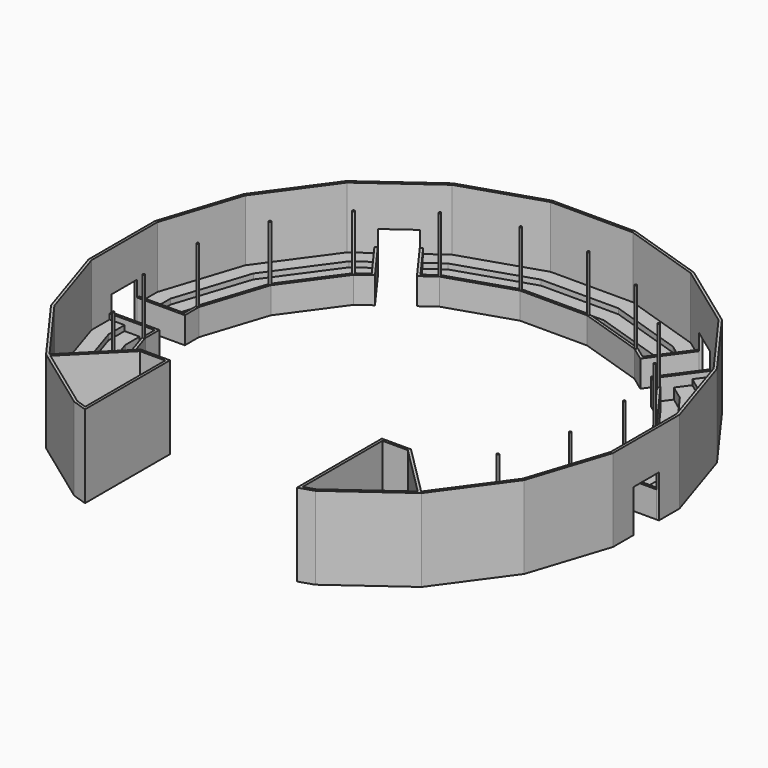
from build123d import *

# Parameters (mm, degrees)
F0_W     = 152.4
F0_H     = 1828.8
F1_DEPTH = 4754.88
F0_R     = 60.96
F2_DEPTH = 1524
F3_DEPTH = 914.4
F4_DEPTH = 1219.2
F5_DEPTH = 304.8
F6_DEPTH = 4724.4
F7_DEPTH = 2438.4


# Not quite as in the source:
# - a feature names something its author has since deleted; it is built from what else it names


with BuildPart() as f1:
    # F0 (on Top) → F1 (new body)
    with BuildSketch(Plane.XY):
        Polygon((2389.6410818405, 15087.6), (-2389.6410818405, 15087.6), (-6935.0085268224, 13610.7205905095), (-8128.5036328315, 12743.5956390277), (-8038.9251603821, 12620.301449085), (-7915.6309704393, 12709.8799215343), (-6864.9579356424, 13473.2385643428), (-2365.503293135, 14935.2), (2365.503293135, 14935.2), (6864.9579356424, 13473.2385643428), (7915.6309704393, 12709.8799215343), (8038.9251603821, 12620.301449085), (8128.5036328314, 12743.5956390277), (6935.0085268224, 13610.7205905095), align=None)
        Polygon((-14935.2, -914.4), (-15087.6, -914.4), (-15087.6, -2389.6410818405), (-13610.7205905095, -6935.0085268224), (-10801.5290181534, -10801.5290181534), (-6935.0085268224, -13610.7205905095), (-6096, -13883.3309861815), (-6096, -7924.8), (-6096, -7772.4), (-6705.6, -7772.4), (-7772.4, -7772.4), (-8728.5082974977, -8728.5082974977), (-8837.6146512164, -8837.6146512164), (-9455.8839889558, -9455.8839889558), (-10074.1533266953, -10074.1533266953), (-10692.4226644347, -10692.4226644347), (-13473.2385643428, -6864.9579356424), (-14935.2, -2365.503293135), (-14935.2, -1066.8), align=None)
        Polygon((-6248.4, -13673.5703815017), (-6864.9579356424, -13473.2385643428), (-10567.5915969054, -10783.117743811), (-7709.2738530943, -7924.8), (-6248.4, -7924.8), align=None, mode=Mode.SUBTRACT)
        Polygon((-14935.2, 914.4), (-15087.6, 914.4), (-15087.6, 0), (-15087.6, -914.4), (-14935.2, -914.4), align=None)
        Polygon((-9565.5489102916, 11511.1443705127), (-9655.127382741, 11634.4385604554), (-10801.5290181534, 10801.5290181534), (-13610.7205905095, 6935.0085268224), (-15087.6, 2389.6410818405), (-15087.6, 914.4), (-14935.2, 914.4), (-14935.2, 1066.8), (-14935.2, 2365.503293135), (-13473.2385643428, 6864.9579356424), (-10692.4226644347, 10692.4226644347), (-9688.8431002343, 11421.5658980633), align=None)
        Polygon((-8038.9251603821, 12620.301449085), (-8128.5036328315, 12743.5956390277), (-9655.127382741, 11634.4385604554), (-9565.5489102916, 11511.1443705127), align=None)
        Polygon((9608.0339121444, 11668.6539696352), (8128.5036328315, 12743.5956390277), (8038.9251603821, 12620.301449085), (9518.455439695, 11545.3597796925), align=None)
        Polygon((10801.5290181534, 10801.5290181534), (9608.0339121444, 11668.6539696352), (9518.455439695, 11545.3597796925), (9641.7496296377, 11455.7813072431), (10692.4226644347, 10692.4226644347), (13473.2385643428, 6864.9579356424), (14935.2, 2365.503293135), (14935.2, 1066.8), (14935.2, 914.4), (15087.6, 914.4), (15087.6, 2389.6410818405), (13610.7205905095, 6935.0085268224), align=None)
        with Locations((15011.4, 0)):
            Rectangle(F0_W, F0_H)
        Polygon((15087.6, -2389.6410818405), (15087.6, -914.4), (14935.2, -914.4), (14935.2, -1066.8), (14935.2, -2365.503293135), (13473.2385643428, -6864.9579356424), (10692.4226644347, -10692.4226644347), (10074.1533266953, -10074.1533266953), (9455.8839889558, -9455.8839889558), (8837.6146512164, -8837.6146512164), (8728.5082974977, -8728.5082974977), (7772.4, -7772.4), (6705.6, -7772.4), (6096, -7772.4), (6096, -13883.3309861815), (6935.0085268224, -13610.7205905095), (10801.5290181534, -10801.5290181534), (13610.7205905095, -6935.0085268224), align=None)
        Polygon((6248.4, -7924.8), (7709.2738530943, -7924.8), (10567.5915969054, -10783.117743811), (6864.9579356424, -13473.2385643428), (6248.4, -13673.5703815017), align=None, mode=Mode.SUBTRACT)
    extrude(amount=F1_DEPTH)

    # F0 (on Top) → F7 (cut)
    with BuildSketch(Plane.XY):
        Polygon((-14935.2, 914.4), (-15087.6, 914.4), (-15087.6, 0), (-15087.6, -914.4), (-14935.2, -914.4), align=None)
        Polygon((-8038.9251603821, 12620.301449085), (-8128.5036328315, 12743.5956390277), (-9655.127382741, 11634.4385604554), (-9565.5489102916, 11511.1443705127), align=None)
        Polygon((9608.0339121444, 11668.6539696352), (8128.5036328315, 12743.5956390277), (8038.9251603821, 12620.301449085), (9518.455439695, 11545.3597796925), align=None)
        with Locations((15011.4, 0)):
            Rectangle(F0_W, F0_H)
    extrude(amount=F7_DEPTH, mode=Mode.SUBTRACT)


with BuildPart() as f2:
    # F0 (on Top) → F2 (new body)
    with BuildSketch(Plane.XY):
        Polygon((-7953.1364062029, 9291.8489515433), (-9565.5489102916, 11511.1443705127), (-9688.8431002343, 11421.5658980633), (-9181.2317563546, 10722.8988217211), (-8673.6204124748, 10024.2317453789), (-8166.009068595, 9325.5646690367), (-8837.6146512164, 8837.6146512164), (-11136.0441195078, 5674.097885582), (-12344.4, 1955.1608851422), (-12344.4, 1066.8), (-13208, 1066.8), (-14071.6, 1066.8), (-14935.2, 1066.8), (-14935.2, 914.4), (-12192, 914.4), (-12192, 1931.0230964367), (-10998.562093341, 5604.047294402), (-8728.5082974977, 8728.5082974977), align=None)
        with Locations((-12268.2, 1943.0919907895)):
            Circle(F0_R, mode=Mode.SUBTRACT)
        with Locations((-11067.3031064244, 5639.072589992)):
            Circle(F0_R, mode=Mode.SUBTRACT)
        with Locations((-8783.0614743571, 8783.0614743571)):
            Circle(F0_R, mode=Mode.SUBTRACT)
    extrude(amount=F2_DEPTH)

    # F0 (on Top) → F3, piece 2 (join)
    with BuildSketch(Plane.XY):
        Polygon((-8673.6204124748, 10024.2317453789), (-9181.2317563546, 10722.8988217211), (-10074.1533266953, 10074.1533266953), (-12694.1737493978, 6468.0045856223), (-14071.6, 2228.7224904707), (-14071.6, 1066.8), (-13208, 1066.8), (-13208, 2091.9416878065), (-11915.1089344528, 6071.0512356021), (-9455.8839889558, 9455.8839889558), align=None)
    extrude(amount=F3_DEPTH)

    # F0 (on Top) → F4 (join)
    with BuildSketch(Plane.XY):
        Polygon((-9181.2317563546, 10722.8988217211), (-9688.8431002343, 11421.5658980633), (-10692.4226644347, 10692.4226644347), (-13473.2385643428, 6864.9579356424), (-14935.2, 2365.503293135), (-14935.2, 1066.8), (-14071.6, 1066.8), (-14071.6, 2228.7224904707), (-12694.1737493978, 6468.0045856223), (-10074.1533266953, 10074.1533266953), align=None)
    extrude(amount=F4_DEPTH)

    # F0 (on Top) → F5, piece 2 (join)
    with BuildSketch(Plane.XY):
        Polygon((-8166.009068595, 9325.5646690367), (-8673.6204124748, 10024.2317453789), (-9455.8839889558, 9455.8839889558), (-11915.1089344528, 6071.0512356021), (-13208, 2091.9416878065), (-13208, 1066.8), (-12344.4, 1066.8), (-12344.4, 1955.1608851422), (-11136.0441195078, 5674.097885582), (-8837.6146512164, 8837.6146512164), align=None)
    extrude(amount=F5_DEPTH)

    # F0 (on Top) → F6, piece 2 (join)
    with BuildSketch(Plane.XY):
        with Locations((-12268.2, 1943.0919907895)):
            Circle(F0_R)
        with Locations((-11067.3031064244, 5639.072589992)):
            Circle(F0_R)
        with Locations((-8783.0614743571, 8783.0614743571)):
            Circle(F0_R)
    extrude(amount=F6_DEPTH)


with BuildPart() as f2b:
    # F0 (on Top) → F2, piece 2 (new body)
    with BuildSketch(Plane.XY):
        Polygon((-7915.6309704393, 12709.8799215343), (-8038.9251603821, 12620.301449085), (-6426.5126562934, 10401.0060301156), (-5604.047294402, 10998.562093341), (-1931.0230964367, 12192), (0, 12192), (0, 12344.4), (-1955.1608851422, 12344.4), (-5674.097885582, 11136.0441195078), (-6392.7969388, 10613.8786925077), (-6900.4082826798, 11312.5457688499), (-7408.0196265596, 12011.2128451921), align=None)
        with Locations((-5639.072589992, 11067.3031064244)):
            Circle(F0_R, mode=Mode.SUBTRACT)
        with Locations((-1943.0919907895, 12268.2)):
            Circle(F0_R, mode=Mode.SUBTRACT)
        Polygon((6426.5126562934, 10401.0060301156), (8038.9251603821, 12620.301449085), (7915.6309704393, 12709.8799215343), (7408.0196265596, 12011.2128451921), (6900.4082826798, 11312.5457688499), (6392.7969388, 10613.8786925077), (5674.097885582, 11136.0441195078), (1955.1608851422, 12344.4), (0, 12344.4), (0, 12192), (1931.0230964367, 12192), (5604.047294402, 10998.562093341), align=None)
        with Locations((5639.072589992, 11067.3031064244)):
            Circle(F0_R, mode=Mode.SUBTRACT)
        with Locations((1943.0919907895, 12268.2)):
            Circle(F0_R, mode=Mode.SUBTRACT)
    extrude(amount=F2_DEPTH)

    # F0 (on Top) → F3, piece 3 (join)
    with BuildSketch(Plane.XY):
        Polygon((-6468.0045856223, 12694.1737493978), (-7408.0196265596, 12011.2128451921), (-6900.4082826798, 11312.5457688499), (-6071.0512356021, 11915.1089344528), (-2091.9416878065, 13208), (2091.9416878065, 13208), (6071.0512356021, 11915.1089344528), (6900.4082826798, 11312.5457688499), (7408.0196265596, 12011.2128451921), (6468.0045856223, 12694.1737493978), (2228.7224904707, 14071.6), (-2228.7224904707, 14071.6), align=None)
    extrude(amount=F3_DEPTH)

    # F0 (on Top) → F4, piece 3 (join)
    with BuildSketch(Plane.XY):
        Polygon((-6864.9579356424, 13473.2385643428), (-7915.6309704393, 12709.8799215343), (-7408.0196265596, 12011.2128451921), (-6468.0045856223, 12694.1737493978), (-2228.7224904707, 14071.6), (2228.7224904707, 14071.6), (6468.0045856223, 12694.1737493978), (7408.0196265596, 12011.2128451921), (7915.6309704393, 12709.8799215343), (6864.9579356424, 13473.2385643428), (2365.503293135, 14935.2), (-2365.503293135, 14935.2), align=None)
    extrude(amount=F4_DEPTH)

    # F0 (on Top) → F5, piece 3 (join)
    with BuildSketch(Plane.XY):
        Polygon((-6071.0512356021, 11915.1089344528), (-6900.4082826798, 11312.5457688499), (-6392.7969388, 10613.8786925077), (-5674.097885582, 11136.0441195078), (-1955.1608851422, 12344.4), (0, 12344.4), (1955.1608851422, 12344.4), (5674.097885582, 11136.0441195078), (6392.7969388, 10613.8786925077), (6900.4082826798, 11312.5457688499), (6071.0512356021, 11915.1089344528), (2091.9416878065, 13208), (-2091.9416878065, 13208), align=None)
    extrude(amount=F5_DEPTH)

    # F0 (on Top) → F6, piece 3 (join)
    with BuildSketch(Plane.XY):
        with Locations((-5639.072589992, 11067.3031064244)):
            Circle(F0_R)
        with Locations((-1943.0919907895, 12268.2)):
            Circle(F0_R)
        with Locations((1943.0919907895, 12268.2)):
            Circle(F0_R)
        with Locations((5639.072589992, 11067.3031064244)):
            Circle(F0_R)
    extrude(amount=F6_DEPTH)


with BuildPart() as f2c:
    # F0 (on Top) → F2, piece 3 (new body)
    with BuildSketch(Plane.XY):
        Polygon((9641.7496296377, 11455.7813072431), (9518.455439695, 11545.3597796925), (7906.0429356063, 9326.0643607231), (8728.5082974977, 8728.5082974977), (10998.562093341, 5604.047294402), (12192, 1931.0230964367), (12192, 914.4), (14935.2, 914.4), (14935.2, 1066.8), (14071.6, 1066.8), (13208, 1066.8), (12344.4, 1066.8), (12344.4, 1955.1608851422), (11136.0441195078, 5674.097885582), (8837.6146512164, 8837.6146512164), (8118.9155979984, 9359.7800782165), (8626.5269418782, 10058.4471545587), (9134.1382857579, 10757.1142309009), align=None)
        with Locations((12268.2, 1943.0919907895)):
            Circle(F0_R, mode=Mode.SUBTRACT)
        with Locations((11067.3031064244, 5639.072589992)):
            Circle(F0_R, mode=Mode.SUBTRACT)
        with Locations((8783.0614743571, 8783.0614743571)):
            Circle(F0_R, mode=Mode.SUBTRACT)
    extrude(amount=F2_DEPTH)

    # F0 (on Top) → F3, piece 4 (join)
    with BuildSketch(Plane.XY):
        Polygon((10074.1533266953, 10074.1533266953), (9134.1382857579, 10757.1142309009), (8626.5269418782, 10058.4471545587), (9455.8839889558, 9455.8839889558), (11915.1089344528, 6071.0512356021), (13208, 2091.9416878065), (13208, 1066.8), (14071.6, 1066.8), (14071.6, 2228.7224904707), (12694.1737493978, 6468.0045856223), align=None)
    extrude(amount=F3_DEPTH)

    # F0 (on Top) → F4, piece 4 (join)
    with BuildSketch(Plane.XY):
        Polygon((10692.4226644347, 10692.4226644347), (9641.7496296377, 11455.7813072431), (9134.1382857579, 10757.1142309009), (10074.1533266953, 10074.1533266953), (12694.1737493978, 6468.0045856223), (14071.6, 2228.7224904707), (14071.6, 1066.8), (14935.2, 1066.8), (14935.2, 2365.503293135), (13473.2385643428, 6864.9579356424), align=None)
    extrude(amount=F4_DEPTH)

    # F0 (on Top) → F5, piece 4 (join)
    with BuildSketch(Plane.XY):
        Polygon((9455.8839889558, 9455.8839889558), (8626.5269418782, 10058.4471545587), (8118.9155979984, 9359.7800782165), (8837.6146512164, 8837.6146512164), (11136.0441195078, 5674.097885582), (12344.4, 1955.1608851422), (12344.4, 1066.8), (13208, 1066.8), (13208, 2091.9416878065), (11915.1089344528, 6071.0512356021), align=None)
    extrude(amount=F5_DEPTH)

    # F0 (on Top) → F6, piece 4 (join)
    with BuildSketch(Plane.XY):
        with Locations((8783.0614743571, 8783.0614743571)):
            Circle(F0_R)
        with Locations((11067.3031064244, 5639.072589992)):
            Circle(F0_R)
        with Locations((12268.2, 1943.0919907895)):
            Circle(F0_R)
    extrude(amount=F6_DEPTH)


with BuildPart() as f2d:
    # F0 (on Top) → F2, piece 4 (new body)
    with BuildSketch(Plane.XY):
        Polygon((-12192, -914.4), (-14935.2, -914.4), (-14935.2, -1066.8), (-14071.6, -1066.8), (-13208, -1066.8), (-12344.4, -1066.8), (-12344.4, -1955.1608851422), (-11136.0441195078, -5674.097885582), (-8837.6146512164, -8837.6146512164), (-8728.5082974977, -8728.5082974977), (-10998.562093341, -5604.047294402), (-12192, -1931.0230964367), align=None)
        with Locations((-11067.3031064244, -5639.072589992)):
            Circle(F0_R, mode=Mode.SUBTRACT)
        with Locations((-12268.2, -1943.0919907895)):
            Circle(F0_R, mode=Mode.SUBTRACT)
    extrude(amount=F2_DEPTH)

    # F0 (on Top) → F3 (join)
    with BuildSketch(Plane.XY):
        Polygon((-13208, -1066.8), (-14071.6, -1066.8), (-14071.6, -2228.7224904707), (-12694.1737493978, -6468.0045856223), (-10074.1533266953, -10074.1533266953), (-9455.8839889558, -9455.8839889558), (-11915.1089344528, -6071.0512356021), (-13208, -2091.9416878065), align=None)
    extrude(amount=F3_DEPTH)

    # F0 (on Top) → F4, piece 2 (join)
    with BuildSketch(Plane.XY):
        Polygon((-14071.6, -1066.8), (-14935.2, -1066.8), (-14935.2, -2365.503293135), (-13473.2385643428, -6864.9579356424), (-10692.4226644347, -10692.4226644347), (-10074.1533266953, -10074.1533266953), (-12694.1737493978, -6468.0045856223), (-14071.6, -2228.7224904707), align=None)
    extrude(amount=F4_DEPTH)

    # F0 (on Top) → F5 (join)
    with BuildSketch(Plane.XY):
        Polygon((-12344.4, -1066.8), (-13208, -1066.8), (-13208, -2091.9416878065), (-11915.1089344528, -6071.0512356021), (-9455.8839889558, -9455.8839889558), (-8837.6146512164, -8837.6146512164), (-11136.0441195078, -5674.097885582), (-12344.4, -1955.1608851422), align=None)
    extrude(amount=F5_DEPTH)

    # F0 (on Top) → F6 (join)
    with BuildSketch(Plane.XY):
        with Locations((-11067.3031064244, -5639.072589992)):
            Circle(F0_R)
        with Locations((-12268.2, -1943.0919907895)):
            Circle(F0_R)
    extrude(amount=F6_DEPTH)


with BuildPart() as f2e:
    # F0 (on Top) → F2, piece 5 (new body)
    with BuildSketch(Plane.XY):
        Polygon((14935.2, -1066.8), (14935.2, -914.4), (12192, -914.4), (12192, -1931.0230964367), (10998.562093341, -5604.047294402), (8728.5082974977, -8728.5082974977), (8837.6146512164, -8837.6146512164), (11136.0441195078, -5674.097885582), (12344.4, -1955.1608851422), (12344.4, -1066.8), (13208, -1066.8), (14071.6, -1066.8), align=None)
        with Locations((11067.3031064244, -5639.072589992)):
            Circle(F0_R, mode=Mode.SUBTRACT)
        with Locations((12268.2, -1943.0919907895)):
            Circle(F0_R, mode=Mode.SUBTRACT)
    extrude(amount=F2_DEPTH)

    # F0 (on Top) → F3, piece 5 (join)
    with BuildSketch(Plane.XY):
        Polygon((14071.6, -2228.7224904707), (14071.6, -1066.8), (13208, -1066.8), (13208, -2091.9416878065), (11915.1089344528, -6071.0512356021), (9455.8839889558, -9455.8839889558), (10074.1533266953, -10074.1533266953), (12694.1737493978, -6468.0045856223), align=None)
    extrude(amount=F3_DEPTH)

    # F0 (on Top) → F4, piece 5 (join)
    with BuildSketch(Plane.XY):
        Polygon((14935.2, -2365.503293135), (14935.2, -1066.8), (14071.6, -1066.8), (14071.6, -2228.7224904707), (12694.1737493978, -6468.0045856223), (10074.1533266953, -10074.1533266953), (10692.4226644347, -10692.4226644347), (13473.2385643428, -6864.9579356424), align=None)
    extrude(amount=F4_DEPTH)

    # F0 (on Top) → F5, piece 5 (join)
    with BuildSketch(Plane.XY):
        Polygon((13208, -2091.9416878065), (13208, -1066.8), (12344.4, -1066.8), (12344.4, -1955.1608851422), (11136.0441195078, -5674.097885582), (8837.6146512164, -8837.6146512164), (9455.8839889558, -9455.8839889558), (11915.1089344528, -6071.0512356021), align=None)
    extrude(amount=F5_DEPTH)

    # F0 (on Top) → F6, piece 5 (join)
    with BuildSketch(Plane.XY):
        with Locations((12268.2, -1943.0919907895)):
            Circle(F0_R)
        with Locations((11067.3031064244, -5639.072589992)):
            Circle(F0_R)
    extrude(amount=F6_DEPTH)


solid = Compound([f1.part, f2.part, f2b.part, f2c.part, f2d.part, f2e.part])
